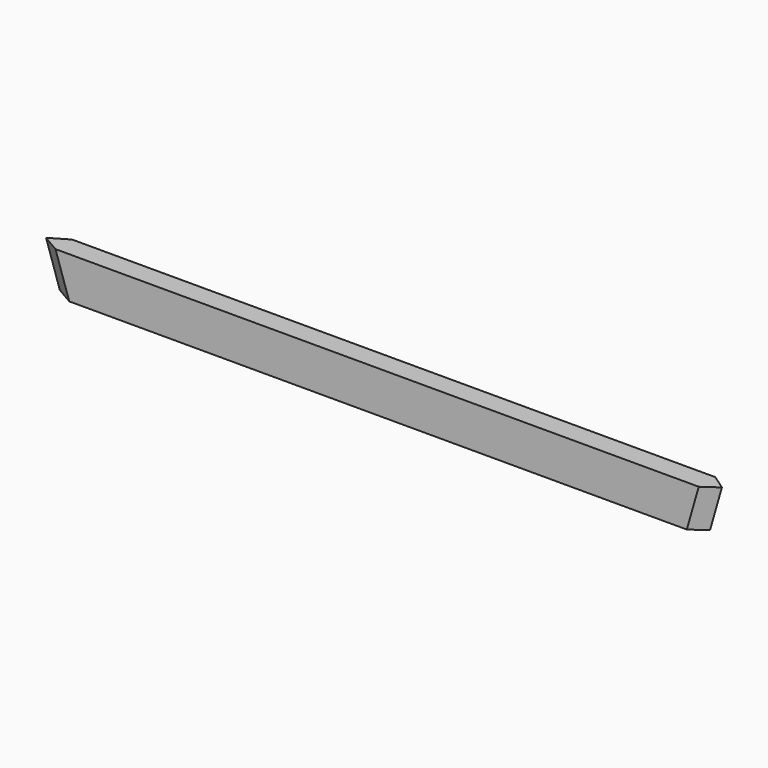
from build123d import *

# Parameters (mm, degrees)
F0_W        = 50
F0_H        = 100
F1_DEPTH    = 819.225
F3_DEPTH    = 50.001
F4_T1_DEPTH = 327.5939866368
F4_T3_DEPTH = 327.5939866368
F5_T1_DEPTH = 329.2426603123
F5_T3_DEPTH = 329.2426603123


# Not quite as in the source:
# - a fillet or chamfer that OpenCascade refuses, or shapes differently, is made with other operations: its cross-section is extruded or revolved along the edge and cut away or added


with BuildPart() as f1:
    # F0 (on Right) → F1 (new body, symmetric)
    with BuildSketch(Plane.YZ):
        Rectangle(F0_W, F0_H)
    extrude(amount=F1_DEPTH, both=True)

    # F2 (on face) → F3 (cut, through all)
    with BuildSketch(Plane.XZ.offset(25)):
        Polygon((819.225, -50), (819.225, 50), (790.5504614241, -50), align=None)
        Polygon((-786.1531619925, -50), (-819.225, 50), (-819.225, -50), align=None)
    extrude(amount=-F3_DEPTH, mode=Mode.SUBTRACT)

    # F4: chamfer of 43.3 x 31.4592914626 on 2 edges, made by hand

    # F4_s2 → F4_t1 (cut)
    with BuildSketch(Plane(origin=(106.3006816601, 0, 370.7145326115), x_dir=(0, 1, 0), z_dir=(-0.2756373558, 0, -0.9612616959))):
        Polygon((-25, 730.4077450642), (6.4592914626, 773.7077450642), (-25, 773.7077450642), align=None)
    extrude(amount=F4_T1_DEPTH, mode=Mode.SUBTRACT)

    # F4_s4 → F4_t3 (cut)
    with BuildSketch(Plane(origin=(16.003541402, 0, 55.8109814378), x_dir=(0, 1, 0), z_dir=(0.2756373558, 0, 0.9612616959))):
        Polygon((-6.4592914626, -773.7077450642), (25, -730.4077450642), (25, -773.7077450642), align=None)
    extrude(amount=F4_T3_DEPTH, mode=Mode.SUBTRACT)

    # F5: chamfer of 43.3 x 26.721749628 on 2 edges, made by hand

    # F5_s2 → F5_t1 (cut)
    with BuildSketch(Plane(origin=(-130.827985574, 0, 395.5872834902), x_dir=(0, 1, 0), z_dir=(0.313992456, 0, -0.9494254776))):
        Polygon((-1.721749628, -762.0934641228), (25, -718.7934641228), (25, -762.0934641228), align=None)
    extrude(amount=F5_T1_DEPTH, mode=Mode.SUBTRACT)

    # F5_s4 → F5_t3 (cut)
    with BuildSketch(Plane(origin=(-27.4482740533, 0, 82.9959134631), x_dir=(0, 1, 0), z_dir=(-0.313992456, 0, 0.9494254776))):
        Polygon((-25, 718.7934641228), (1.721749628, 762.0934641228), (-25, 762.0934641228), align=None)
    extrude(amount=F5_T3_DEPTH, mode=Mode.SUBTRACT)


solid = f1.part
